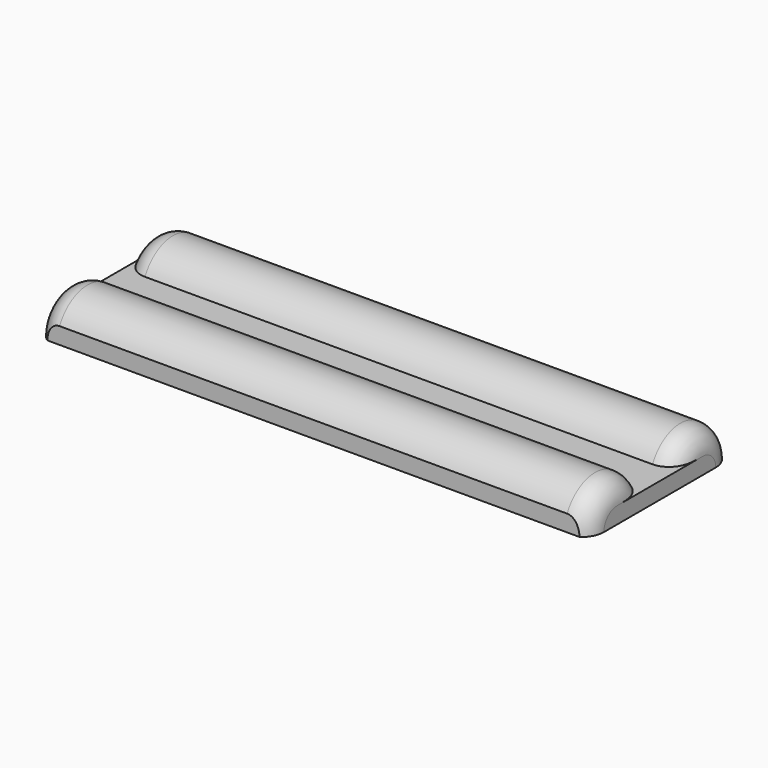
from build123d import *

# Parameters (mm, degrees)
F0_W     = 50
F0_H     = 16
F1_DEPTH = 1.5
F3_DEPTH = 50
F4_R     = 1.99999


# Not quite as in the source:
# - a fillet or chamfer is up to 0.001 mm smaller than in the source, because OpenCascade refuses the exact size


with BuildPart() as f1:
    # F0 (on Top) → F1 (new body)
    with BuildSketch(Plane.XY):
        Rectangle(F0_W, F0_H)
    extrude(amount=-F1_DEPTH)

    # F2 (on face) → F3 (join)
    with BuildSketch(Plane(origin=(-25, 0, 0), x_dir=(0, -1, 0), z_dir=(-1, 0, 0))):
        with BuildLine():
            ThreePointArc((-1.6754446797, 0), (-4.8377223398, 2), (-8, 0))
            Line((-8, 0), (-1.6754446797, 0))
        make_face()
        with BuildLine():
            ThreePointArc((8, 0), (4.8377223398, 2), (1.6754446797, 0))
            Line((1.6754446797, 0), (8, 0))
        make_face()
    extrude(amount=-F3_DEPTH)

    # F4 (radius 2 in the source; OpenCascade refuses exactly that, so slightly less here)
    f4_edges = [f1.edges().sort_by_distance(p)[0] for p in [
        (-25, -4.837722, 2),
        (-25, 4.837722, 2),
        (25, -4.837722, 2),
        (25, 4.837722, 2),
    ]]
    fillet(f4_edges, radius=F4_R)


solid = f1.part
